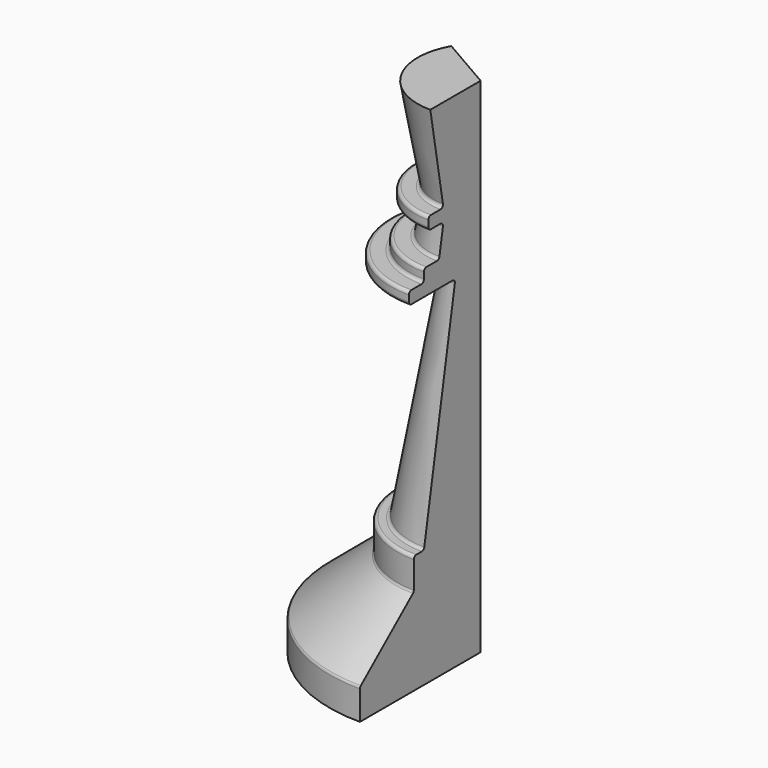
from build123d import *

# Parameters (mm, degrees)
F1_ANGLE_BACK = 30
F1_ANGLE      = 120


# Not quite as in the source:
# - a feature of the source that left no trace in its solid (it failed there, or was rolled back) is left out


with BuildPart() as f1:
    # F0 (on Front) → F1 (revolve)
    with BuildSketch(Plane.XZ, mode=Mode.PRIVATE) as f1_sk:
        with BuildLine():
            Line((-15.24, 0), (0, 0))
            Line((0, 0), (0, 50.8))
            Line((0, 50.8), (-6.35, 50.8))
            Line((-6.35, 50.8), (-4.7617064118, 41.792339449))
            ThreePointArc((-4.7617064118, 41.792339449), (-4.8311637627, 41.5331210865), (-5.0743828734, 41.4197061526))
            Line((-5.0743828734, 41.4197061526), (-6.2835011077, 41.4197061526))
            ThreePointArc((-6.2835011077, 41.4197061526), (-6.5080075107, 41.3267125556), (-6.6010011077, 41.1022061526))
            Line((-6.6010011077, 41.1022061526), (-6.6010011077, 40.4672061526))
            ThreePointArc((-6.6010011077, 40.4672061526), (-6.5080075107, 40.2426997495), (-6.2835011077, 40.1497061526))
            Line((-6.2835011077, 40.1497061526), (-5.0743828734, 40.1497061526))
            ThreePointArc((-5.0743828734, 40.1497061526), (-4.8311637627, 40.0362912186), (-4.7617064118, 39.7770728561))
            Line((-4.7617064118, 39.7770728561), (-5.2010717431, 37.2853082403))
            ThreePointArc((-5.2010717431, 37.2853082403), (-5.3096631386, 37.0972224261), (-5.5137482047, 37.0229415367))
            Line((-5.5137482047, 37.0229415367), (-6.8348340718, 37.0229415367))
            ThreePointArc((-6.8348340718, 37.0229415367), (-7.0593404748, 36.9299479398), (-7.1523340718, 36.7054415367))
            Line((-7.1523340718, 36.7054415367), (-7.1523340718, 36.0704415367))
            ThreePointArc((-7.1523340718, 36.0704415367), (-7.2453276688, 35.8459351337), (-7.4698340718, 35.7529415367))
            Line((-7.4698340718, 35.7529415367), (-8.7398340718, 35.7529415367))
            ThreePointArc((-8.7398340718, 35.7529415367), (-8.9643404748, 35.6599479398), (-9.0573340718, 35.4354415367))
            Line((-9.0573340718, 35.4354415367), (-9.0573340718, 34.8004415367))
            ThreePointArc((-9.0573340718, 34.8004415367), (-8.9643404748, 34.5759351337), (-8.7398340718, 34.4829415367))
            Line((-8.7398340718, 34.4829415367), (-3.5686493249, 34.4829415367))
            ThreePointArc((-3.5686493249, 34.4829415367), (-3.3254302142, 34.3695266028), (-3.2559728633, 34.1103082403))
            Line((-3.2559728633, 34.1103082403), (-7.113602572, 12.2326030065))
            ThreePointArc((-7.113602572, 12.2326030065), (-7.2221939675, 12.0445171922), (-7.4262790336, 11.9702363029))
            Line((-7.4262790336, 11.9702363029), (-8.1123649007, 11.9702363029))
            ThreePointArc((-8.1123649007, 11.9702363029), (-8.3368713037, 11.8772427059), (-8.4298649007, 11.6527363029))
            Line((-8.4298649007, 11.6527363029), (-8.4298649007, 8.9432889844))
            ThreePointArc((-8.4298649007, 8.9432889844), (-8.4596121783, 8.8091076862), (-8.5432798346, 8.7000698737))
            Line((-8.5432798346, 8.7000698737), (-15.1265850661, 3.176020882))
            ThreePointArc((-15.1265850661, 3.176020882), (-15.2102527224, 3.0669830694), (-15.24, 2.9328017713))
            Line((-15.24, 2.9328017713), (-15.24, 0))
        make_face()
    revolve(f1_sk.sketch.rotate(Axis((0, 0, 25.4), (0, 0, 1)), -F1_ANGLE_BACK), axis=Axis((0, 0, 25.4), (0, 0, 1)), revolution_arc=F1_ANGLE)


solid = f1.part
